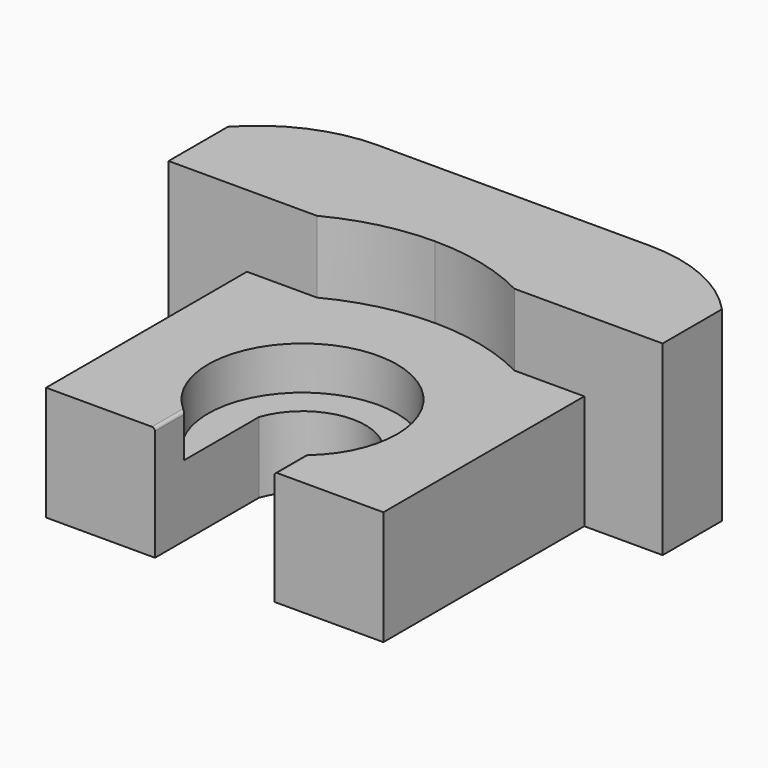
from build123d import *

# Parameters (mm, degrees)
F1_DEPTH = 2.35
F2_DEPTH = 3.78
F3_DEPTH = 6.16
F4_R     = 0.1
F5_R     = 0.1


# Not quite as in the source:
# - a feature names something its author has since deleted; it is built from what else it names


with BuildPart() as f1:
    # F0 (on Top) → F1 (new body)
    with BuildSketch(Plane.XY):
        with BuildLine():
            Line((0.6766474014, -1.6654146139), (0.6766474014, -4.7543960131))
            ThreePointArc((0.6766474014, -4.7543960131), (1.524544849, -3.6730954673), (1.8266474014, -2.3326198054))
            ThreePointArc((1.8266474014, -2.3326198054), (-2.6388282605, 0.4902776422), (-3.2733525986, -4.7543960131))
            Line((-3.2733525986, -4.7543960131), (-3.2733525986, -1.6654146139))
            ThreePointArc((-3.2733525986, -1.6654146139), (-1.2983525986, -0.247964494), (0.6766474014, -1.6654146139))
        make_face()
    extrude(amount=F1_DEPTH)

    # F0 (on Top) → F2 (join)
    with BuildSketch(Plane.XY):
        with BuildLine():
            Line((4.2766474014, -5.9583943095), (4.2766474014, 2.3416056905))
            Line((4.2766474014, 2.3416056905), (1.9666474014, 2.3416056905))
            ThreePointArc((1.9666474014, 2.3416056905), (0.3815359204, 2.9330616855), (-1.2983525986, 3.1339924307))
            ThreePointArc((-1.2983525986, 3.1339924307), (-2.9782411177, 2.9330616855), (-4.5633525986, 2.3416056905))
            Line((-4.5633525986, 2.3416056905), (-6.8733525986, 2.3416056905))
            Line((-6.8733525986, 2.3416056905), (-6.8733525986, -5.9583943095))
            Line((-6.8733525986, -5.9583943095), (-3.2733525986, -5.9583943095))
            Line((-3.2733525986, -5.9583943095), (-3.2733525986, -4.7543960131))
            ThreePointArc((-3.2733525986, -4.7543960131), (-2.6388282605, 0.4902776422), (1.8266474014, -2.3326198054))
            ThreePointArc((1.8266474014, -2.3326198054), (1.524544849, -3.6730954673), (0.6766474014, -4.7543960131))
            Line((0.6766474014, -4.7543960131), (0.6766474014, -5.9583943095))
            Line((0.6766474014, -5.9583943095), (4.2766474014, -5.9583943095))
        make_face()
    extrude(amount=F2_DEPTH)

    # F0 (on Top) → F3 (join)
    with BuildSketch(Plane.XY):
        with BuildLine():
            ThreePointArc((-4.5633525986, 2.3416056905), (-2.9782411177, 2.9330616855), (-1.2983525986, 3.1339924307))
            Line((-1.2983525986, 3.1339924307), (-1.2983525986, 4.7916056905))
            Line((-1.2983525986, 4.7916056905), (-9.4633525986, 4.7916056905))
            Line((-9.4633525986, 4.7916056905), (-9.4633525986, 2.3416056905))
            Line((-9.4633525986, 2.3416056905), (-6.8733525986, 2.3416056905))
            Line((-6.8733525986, 2.3416056905), (-4.5633525986, 2.3416056905))
        make_face()
        with BuildLine():
            Line((1.9666474014, 2.3416056905), (4.2766474014, 2.3416056905))
            Line((4.2766474014, 2.3416056905), (6.8666474014, 2.3416056905))
            Line((6.8666474014, 2.3416056905), (6.8666474014, 4.7916056905))
            Line((6.8666474014, 4.7916056905), (-1.2983525986, 4.7916056905))
            Line((-1.2983525986, 4.7916056905), (-1.2983525986, 3.1339924307))
            ThreePointArc((-1.2983525986, 3.1339924307), (0.3815359204, 2.9330616855), (1.9666474014, 2.3416056905))
        make_face()
        with BuildLine():
            Line((-1.2983525986, 4.7916056905), (6.8666474014, 4.7916056905))
            ThreePointArc((6.8666474014, 4.7916056905), (5.2036474014, 5.9830772848), (3.2016474014, 6.4039924307))
            Line((3.2016474014, 6.4039924307), (-1.2983525986, 6.4039924307))
            Line((-1.2983525986, 6.4039924307), (-1.2983525986, 4.7916056905))
        make_face()
        with BuildLine():
            Line((-9.4633525986, 4.7916056905), (-1.2983525986, 4.7916056905))
            Line((-1.2983525986, 4.7916056905), (-1.2983525986, 6.4039924307))
            Line((-1.2983525986, 6.4039924307), (-5.7983525986, 6.4039924307))
            ThreePointArc((-5.7983525986, 6.4039924307), (-7.8003525986, 5.9830772848), (-9.4633525986, 4.7916056905))
        make_face()
    extrude(amount=F3_DEPTH)

    # F4
    f4_edges = [f1.edges().sort_by_distance(p)[0] for p in [
        (0.676647, -5.356395, 3.78),
    ]]
    fillet(f4_edges, radius=F4_R)

    # F5
    f5_edges = [f1.edges().sort_by_distance(p)[0] for p in [
        (-3.273353, -5.356395, 3.78),
    ]]
    fillet(f5_edges, radius=F5_R)


solid = f1.part
